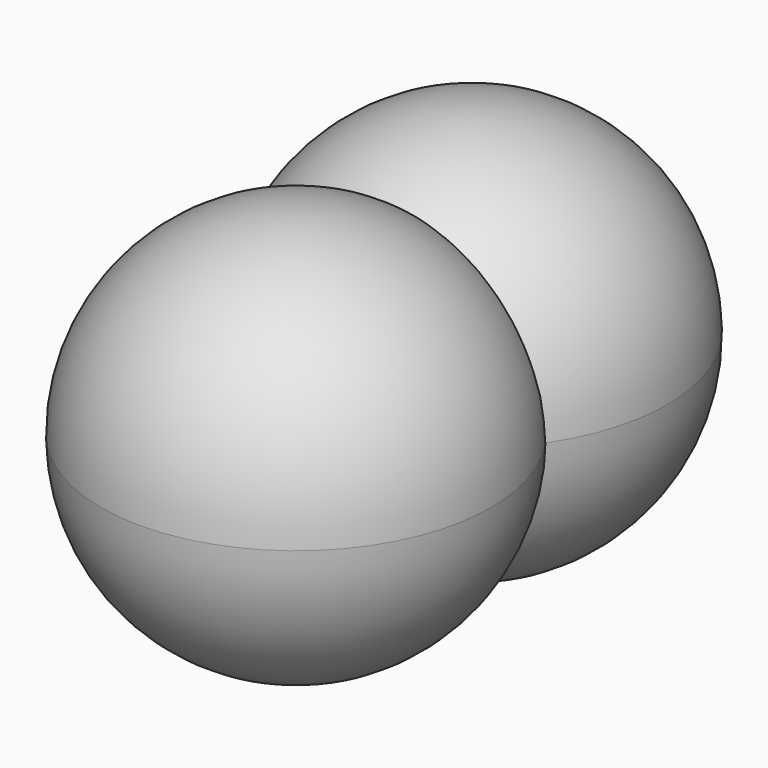
from build123d import *

# Parameters (mm, degrees)
F4_SCALE = 0.5


with BuildPart() as f1:
    # F0 (on Right) → F1 (revolve)
    with BuildSketch(Plane.YZ):
        with BuildLine():
            ThreePointArc((3.81, 0), (2.6940768363, 2.6940768363), (0, 3.81))
            Line((0, 3.81), (0, -3.81))
            ThreePointArc((0, -3.81), (2.6940768363, -2.6940768363), (3.81, 0))
        make_face()
    revolve(axis=Axis((0, 0, -1.8932370985), (0, 0, -1)))


with BuildPart() as f3:
    # F2 (on Right) → F3 (revolve)
    with BuildSketch(Plane.YZ):
        with BuildLine():
            ThreePointArc((8.1009025215, 0.0203915406), (6.9849793578, 2.7144683769), (4.2909025215, 3.8303915406))
            Line((4.2909025215, 3.8303915406), (4.2909025215, -3.7896084594))
            ThreePointArc((4.2909025215, -3.7896084594), (6.9849793578, -2.6736852957), (8.1009025215, 0.0203915406))
        make_face()
    revolve(axis=Axis((0, 4.2909025215, 0.0203915406), (0, 0, -1)))


with BuildPart() as f3_1:
    # F4: moved
    add(f3.part.scale(F4_SCALE))


with BuildPart() as f1_1:
    # F4: moved
    add(f1.part.scale(F4_SCALE))


solid = Compound([f3_1.part, f1_1.part])
